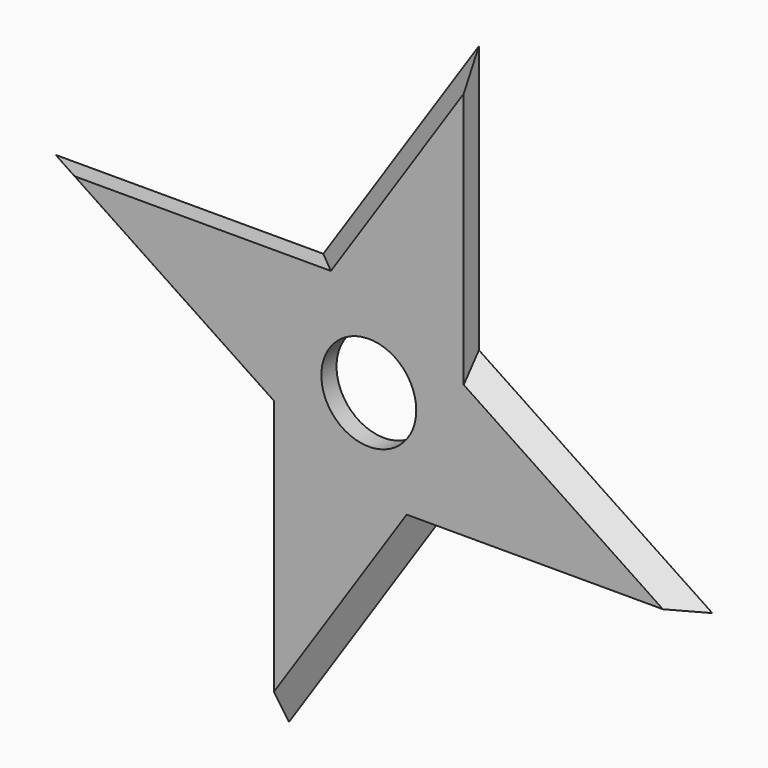
from build123d import *

# Parameters (mm, degrees)
F0_R         = 5
F1_DEPTH     = 2
F2_T4_DEPTH  = 61.7723426343
F2_T9_DEPTH  = 61.7723426343
F2_T14_DEPTH = 61.7723426343
F2_T19_DEPTH = 61.7723426343


# Not quite as in the source:
# - a fillet or chamfer that OpenCascade refuses, or shapes differently, is made with other operations: its cross-section is extruded or revolved along the edge and cut away or added


with BuildPart() as f1:
    # F0 (on Front) → F1 (new body)
    with BuildSketch(Plane.XZ):
        Polygon((10, 40), (-10, 10), (-40, 10), (-10, -10), (-10, -40), (10, -10), (40, -10), (10, 10), align=None)
        Circle(F0_R, mode=Mode.SUBTRACT)
    extrude(amount=F1_DEPTH)

    # F2: chamfer of 5 on 4 edges, made by hand


with BuildPart() as f2_tool2:
    # F2_s3 → F2_t4 (new body)
    with BuildSketch(Plane(origin=(43.0065402431, 0, -28.6710268287), x_dir=(0, 1, 0), z_dir=(-0.8320502943, 0, 0.5547001962))):
        Polygon((3, -13.8675049056), (-2, -8.8675049056), (-2, -13.8675049056), align=None)
    extrude(amount=F2_T4_DEPTH)

    split(bisect_by=Plane.YZ.offset(10), keep=Keep.TOP)


with BuildPart() as f1_1:
    add(f1.part)

    # F2_t1: cut F2_tool2
    add(f2_tool2.part, mode=Mode.SUBTRACT)


with BuildPart() as f2_tool7:
    # F2_s8 → F2_t9 (new body)
    with BuildSketch(Plane(origin=(28.6710268287, 0, 43.0065402431), x_dir=(0, 1, 0), z_dir=(-0.5547001962, 0, -0.8320502943))):
        Polygon((3, -13.8675049056), (-2, -8.8675049056), (-2, -13.8675049056), align=None)
    extrude(amount=F2_T9_DEPTH)

    split(bisect_by=Plane.XY.offset(10), keep=Keep.TOP)


with BuildPart() as f1_2:
    add(f1_1.part)

    # F2_t6: cut F2_tool7
    add(f2_tool7.part, mode=Mode.SUBTRACT)


with BuildPart() as f2_tool12:
    # F2_s13 → F2_t14 (new body)
    with BuildSketch(Plane(origin=(-43.0065402431, 0, 28.6710268287), x_dir=(0, 1, 0), z_dir=(0.8320502943, 0, -0.5547001962))):
        Polygon((3, -13.8675049056), (-2, -8.8675049056), (-2, -13.8675049056), align=None)
    extrude(amount=F2_T14_DEPTH)

    split(bisect_by=Plane.YZ.offset(-10), keep=Keep.BOTTOM)


with BuildPart() as f1_3:
    add(f1_2.part)

    # F2_t11: cut F2_tool12
    add(f2_tool12.part, mode=Mode.SUBTRACT)


with BuildPart() as f2_tool17:
    # F2_s18 → F2_t19 (new body)
    with BuildSketch(Plane(origin=(-28.6710268287, 0, -43.0065402431), x_dir=(0, 1, 0), z_dir=(0.5547001962, 0, 0.8320502943))):
        Polygon((3, -13.8675049056), (-2, -8.8675049056), (-2, -13.8675049056), align=None)
    extrude(amount=F2_T19_DEPTH)

    split(bisect_by=Plane.XY.offset(-10), keep=Keep.BOTTOM)


with BuildPart() as f1_4:
    add(f1_3.part)

    # F2_t16: cut F2_tool17
    add(f2_tool17.part, mode=Mode.SUBTRACT)


solid = f1_4.part
